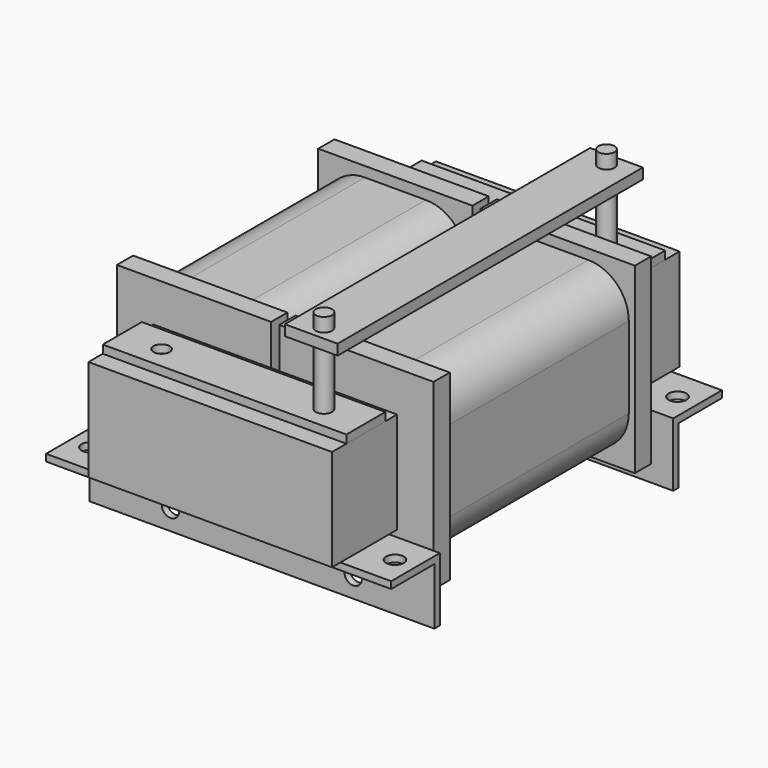
from build123d import *

# Parameters (mm, degrees)
F0_W           = 20
F0_H           = 25
F1_DEPTH       = 28.5
F2_W           = 38
F2_H           = 45
F3_DEPTH       = 5
F6_W           = 29
F6_H           = 25
F6_W_2         = 31
F7_DEPTH       = 20
F9_W           = 60
F9_H           = 12
F9_R           = 2
F10_DEPTH      = 2
F12_W          = 12.5
F12_H          = 1.7
F12_H_2        = 13.3
F12_R          = 2.18
F12_W_2        = 60
F13_DEPTH      = 1.7
F14_W          = 85
F14_H          = 1.7
F15_DEPTH      = 14
F16_R          = 2.15
F17_DEPTH      = 1.7
F20_W          = 13
F20_H          = 94
F21_DEPTH      = 2.6
F22_DEPTH      = 23
F22_DEPTH_BACK = 27


with BuildPart() as f1:
    # F0 (on Front) → F1 (new body, symmetric)
    with BuildSketch(Plane.XZ):
        with Locations((-20, 0)):
            Rectangle(F0_W, F0_H)
        with BuildLine():
            ThreePointArc((-12.5, -20), (-6.376275643, -17.9056941504), (-2.8175416345, -12.5))
            Line((-2.8175416345, -12.5), (-10, -12.5))
            Line((-10, -12.5), (-30, -12.5))
            Line((-30, -12.5), (-30, 12.5))
            Line((-30, 12.5), (-10, 12.5))
            Line((-10, 12.5), (-2.8175416345, 12.5))
            ThreePointArc((-2.8175416345, 12.5), (-6.376275643, 17.9056941504), (-12.5, 20))
            Line((-12.5, 20), (-27.5, 20))
            ThreePointArc((-27.5, 20), (-34.5710678119, 17.0710678119), (-37.5, 10))
            Line((-37.5, 10), (-37.5, -10))
            ThreePointArc((-37.5, -10), (-34.5710678119, -17.0710678119), (-27.5, -20))
            Line((-27.5, -20), (-12.5, -20))
        make_face()
        with BuildLine():
            Line((-10, -12.5), (-2.8175416345, -12.5))
            ThreePointArc((-2.8175416345, -12.5), (-2.5797030373, -11.2600429248), (-2.5, -10))
            Line((-2.5, -10), (-2.5, 10))
            ThreePointArc((-2.5, 10), (-2.5797030373, 11.2600429248), (-2.8175416345, 12.5))
            Line((-2.8175416345, 12.5), (-10, 12.5))
            Line((-10, 12.5), (-10, -12.5))
        make_face()
    extrude(amount=F1_DEPTH, both=True)


with BuildPart() as f1b:
    # F0 (on Front) → F1, piece 2 (new body, symmetric)
    with BuildSketch(Plane.XZ):
        with Locations((20, 0)):
            Rectangle(F0_W, F0_H)
        with BuildLine():
            Line((2.8175416345, -12.5), (10, -12.5))
            Line((10, -12.5), (10, 12.5))
            Line((10, 12.5), (2.8175416345, 12.5))
            ThreePointArc((2.8175416345, 12.5), (2.5797030373, 11.2600429248), (2.5, 10))
            Line((2.5, 10), (2.5, -10))
            ThreePointArc((2.5, -10), (2.5797030373, -11.2600429248), (2.8175416345, -12.5))
        make_face()
        with BuildLine():
            Line((30, 12.5), (30, -12.5))
            Line((30, -12.5), (10, -12.5))
            Line((10, -12.5), (2.8175416345, -12.5))
            ThreePointArc((2.8175416345, -12.5), (6.376275643, -17.9056941504), (12.5, -20))
            Line((12.5, -20), (27.5, -20))
            ThreePointArc((27.5, -20), (34.5710678119, -17.0710678119), (37.5, -10))
            Line((37.5, -10), (37.5, 10))
            ThreePointArc((37.5, 10), (34.5710678119, 17.0710678119), (27.5, 20))
            Line((27.5, 20), (12.5, 20))
            ThreePointArc((12.5, 20), (6.376275643, 17.9056941504), (2.8175416345, 12.5))
            Line((2.8175416345, 12.5), (10, 12.5))
            Line((10, 12.5), (30, 12.5))
        make_face()
    extrude(amount=F1_DEPTH, both=True)


with BuildPart() as f3:
    # F2 (on face) → F3 (new body)
    with BuildSketch(Plane.XZ.offset(28.5)):
        with Locations((-20, 0)):
            Rectangle(F2_W, F2_H)
        with BuildLine():
            Line((-27.5, 20), (-12.5, 20))
            ThreePointArc((-12.5, 20), (-5.4289321881, 17.0710678119), (-2.5, 10))
            Line((-2.5, 10), (-2.5, -10))
            ThreePointArc((-2.5, -10), (-5.4289321881, -17.0710678119), (-12.5, -20))
            Line((-12.5, -20), (-27.5, -20))
            ThreePointArc((-27.5, -20), (-34.5710678119, -17.0710678119), (-37.5, -10))
            Line((-37.5, -10), (-37.5, 10))
            ThreePointArc((-37.5, 10), (-34.5710678119, 17.0710678119), (-27.5, 20))
        make_face(mode=Mode.SUBTRACT)
        with BuildLine():
            ThreePointArc((-2.5, 10), (-5.4289321881, 17.0710678119), (-12.5, 20))
            Line((-12.5, 20), (-27.5, 20))
            ThreePointArc((-27.5, 20), (-34.5710678119, 17.0710678119), (-37.5, 10))
            Line((-37.5, 10), (-37.5, -10))
            ThreePointArc((-37.5, -10), (-34.5710678119, -17.0710678119), (-27.5, -20))
            Line((-27.5, -20), (-12.5, -20))
            ThreePointArc((-12.5, -20), (-5.4289321881, -17.0710678119), (-2.5, -10))
            Line((-2.5, -10), (-2.5, 10))
        make_face()
    extrude(amount=F3_DEPTH)


with BuildPart() as f4_1:
    # F4: instance of F3
    add(f3.part.mirror(Plane.YZ))


with BuildPart() as f5_1:
    # F5: instance of F3
    add(f3.part.mirror(Plane.XZ))


with BuildPart() as f5_2:
    # F5: instance of F4_1
    add(f4_1.part.mirror(Plane.XZ))


with BuildPart() as f7:
    # F6 (on face) → F7 (new body)
    with BuildSketch(Plane.XZ.offset(33.5)):
        with Locations((-15.5, 0)):
            Rectangle(F6_W, F6_H)
        with Locations((14.5, 0)):
            Rectangle(F6_W_2, F6_H)
    extrude(amount=F7_DEPTH)


with BuildPart() as f8_1:
    # F8: instance of F7
    add(f7.part.mirror(Plane.XZ))


with BuildPart() as f10:
    # F9 (on face) → F10 (new body)
    with BuildSketch(Plane.XY.offset(12.5)):
        with Locations((0, -43.0828370154)):
            Rectangle(F9_W, F9_H)
        with Locations((-20, -43.5)):
            Circle(F9_R, mode=Mode.SUBTRACT)
        with Locations((20, -43.5)):
            Circle(F9_R, mode=Mode.SUBTRACT)
    extrude(amount=F10_DEPTH)


with BuildPart() as f11_1:
    # F11: instance of F10
    add(f10.part.mirror(Plane.XZ))


with BuildPart() as f13:
    # F12 (on face) → F13 (new body)
    with BuildSketch(Plane(origin=(0, 0, -12.5), x_dir=(1, 0, 0), z_dir=(0, 0, -1))):
        with Locations((-36.25, 36.774602598)):
            Rectangle(F12_W, F12_H)
        with Locations((-36.25, 44.274602598)):
            Rectangle(F12_W, F12_H_2)
        with Locations((-37.5, 43.5)):
            Circle(F12_R, mode=Mode.SUBTRACT)
        with Locations((36.25, 36.774602598)):
            Rectangle(F12_W, F12_H)
        with Locations((36.25, 44.274602598)):
            Rectangle(F12_W, F12_H_2)
        with Locations((37.5, 43.5)):
            Circle(F12_R, mode=Mode.SUBTRACT)
        with Locations((0, 36.774602598)):
            Rectangle(F12_W_2, F12_H)
        with Locations((0, 44.274602598)):
            Rectangle(F12_W_2, F12_H_2)
    extrude(amount=F13_DEPTH)

    # F14 (on face) → F15 (join)
    with BuildSketch(Plane(origin=(0, 0, -14.2), x_dir=(1, 0, 0), z_dir=(0, 0, -1))):
        with Locations((0, 36.774602598)):
            Rectangle(F14_W, F14_H)
    extrude(amount=F15_DEPTH)

    # F16 (on face) → F17 (cut, through all)
    with BuildSketch(Plane.XZ.offset(37.624602598)):
        with Locations((-22.5, -23.2)):
            Circle(F16_R)
        with Locations((22.5, -23.2)):
            Circle(F16_R)
    extrude(amount=-F17_DEPTH, mode=Mode.SUBTRACT)


with BuildPart() as f18_1:
    # F18: instance of F13
    add(f13.part.mirror(Plane.XZ))


with BuildPart() as f21:
    # F20 (on offset) → F21 (new body)
    with BuildSketch(Plane.XY.offset(29.5)):
        with Locations((19.6661213413, 0)):
            Rectangle(F20_W, F20_H)
    extrude(amount=F21_DEPTH)


with BuildPart() as f22:
    # F9 (on face) → F22 (new body, two sides)
    with BuildSketch(Plane.XY.offset(12.5)) as f22_sk:
        with Locations((20, -43.5)):
            Circle(F9_R)
    extrude(amount=F22_DEPTH)
    extrude(f22_sk.sketch, amount=-F22_DEPTH_BACK)


with BuildPart() as f23_1:
    # F23: instance of F22
    add(f22.part.mirror(Plane.XZ))


solid = Compound([f1.part, f1b.part, f3.part, f4_1.part, f5_1.part, f5_2.part, f7.part, f8_1.part, f10.part, f11_1.part, f13.part, f18_1.part, f21.part, f22.part, f23_1.part])
